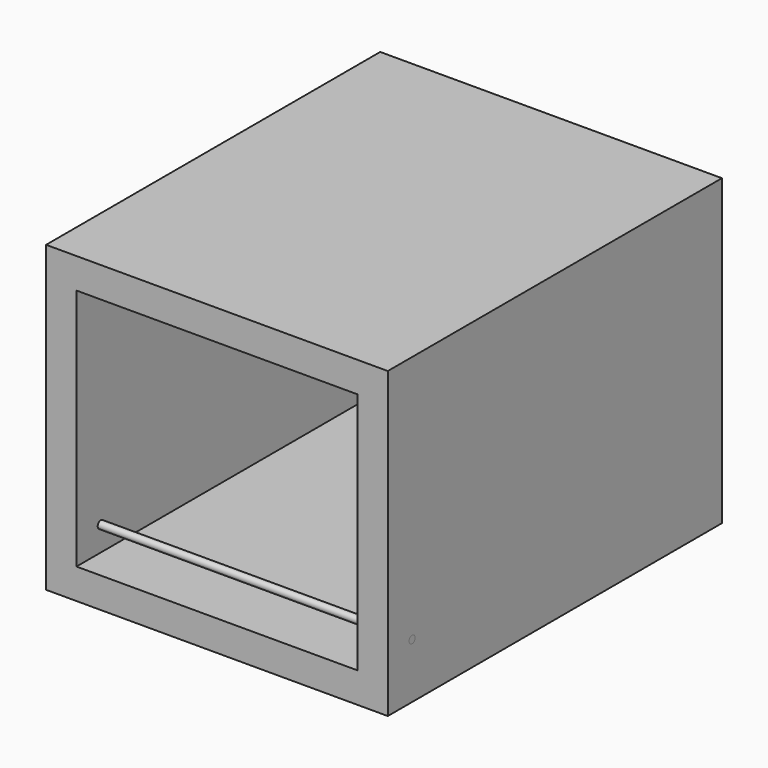
from build123d import *

# Parameters (mm, degrees)
F0_W     = 45
F0_H     = 102
F0_H_2   = 8
F1_DEPTH = 80
F2_T     = -8


# Not quite as in the source:
# - a feature names something its author has since deleted; it is built from what else it names


with BuildPart() as f1:
    # F0 (on Top) → F1 (new body)
    with BuildSketch(Plane.XY):
        with Locations((-22.5, 10.8258862279)):
            Rectangle(F0_W, F0_H)
        with Locations((22.5, 10.8258862279)):
            Rectangle(F0_W, F0_H)
        with Locations((22.5, -44.1741137721)):
            Rectangle(F0_W, F0_H_2)
        with Locations((-22.5, -44.1741137721)):
            Rectangle(F0_W, F0_H_2)
    extrude(amount=F1_DEPTH)

    # F2
    f2_openings = [f1.faces().sort_by_distance(p)[0] for p in [
        (0, -48.174114, 40),
    ]]
    offset(amount=F2_T, openings=f2_openings)


with BuildPart() as f6:
    # F5 (on 3pt) → F6 (revolve)
    with BuildSketch(Plane(origin=(4.3298e-06, -40.17411, 0), x_dir=(1, 1.078e-07, 0), z_dir=(1.078e-07, -1, 0))):
        Polygon((-45, 13.5), (0, 13.5), (45, 13.5), (45, 14.5), (0, 14.5), (-45, 14.5), align=None)
    revolve(axis=Axis((22.5000043298, -40.174107575, 14.5), (1, 1.078e-07, 0)))


solid = Compound([f1.part, f6.part])
